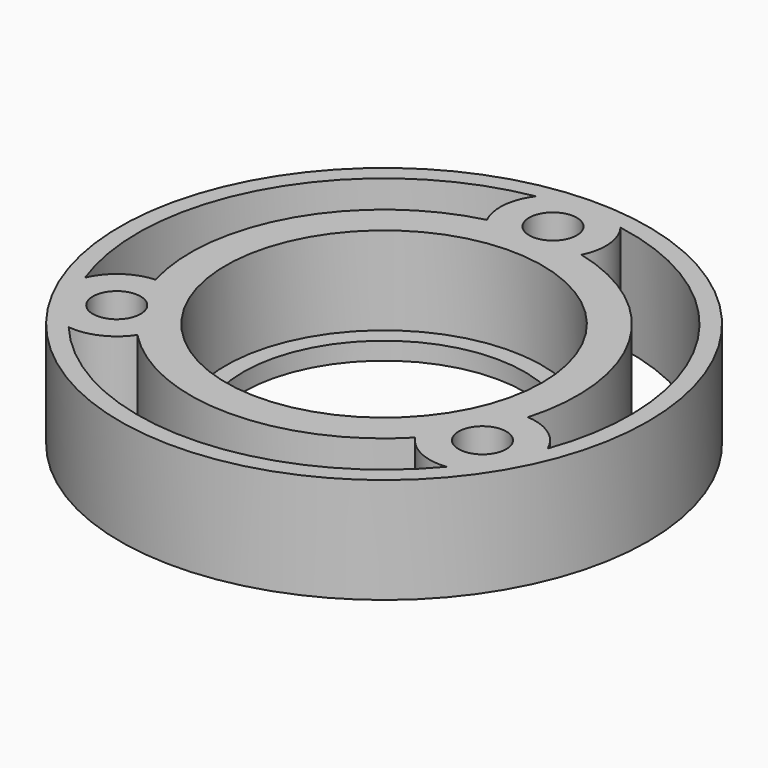
from build123d import *

# Parameters (mm, degrees)
F0_R            = 23.8125
F0_R_2          = 2.15265
F0_R_3          = 12.7
F1_DEPTH        = 9.525
F2_R            = 14.2875
F3_DEPTH        = 7.9375
F5_DEPTH        = 9.525
F5_COPIES_COUNT = 3


# Not quite as in the source:
# - a pattern or mirror of a feature is missing from the dataset's text; its kind, count and spacing are read off the source's solid


with BuildPart() as f1:
    # F0 (on Top) → F1 (new body)
    with BuildSketch(Plane.XY):
        Circle(F0_R)
        with Locations((-16.4977839421, -9.525)):
            Circle(F0_R_2, mode=Mode.SUBTRACT)
        with Locations((16.4977839421, -9.525)):
            Circle(F0_R_2, mode=Mode.SUBTRACT)
        Circle(F0_R_3, mode=Mode.SUBTRACT)
        with Locations((0, 19.05)):
            Circle(F0_R_2, mode=Mode.SUBTRACT)
    extrude(amount=F1_DEPTH)

    # F2 (on face) → F3 (cut)
    with BuildSketch(Plane.XY.offset(9.525)):
        Circle(F2_R)
    extrude(amount=-F3_DEPTH, mode=Mode.SUBTRACT)

    # F4 (on face) → F5 (cut, through all)
    with BuildSketch(Plane.XY.offset(9.525)):
        with BuildLine():
            ThreePointArc((17.0510516982, -14.2552538029), (14.4957458217, -13.8462555599), (12.5315578082, -12.1613718449))
            ThreePointArc((12.5315578082, -12.1613718449), (0, -17.4625), (-12.5315578082, -12.1613718449))
            ThreePointArc((-12.5315578082, -12.1613718449), (-14.4957458217, -13.8462555599), (-17.0510516982, -14.2552538029))
            ThreePointArc((-17.0510516982, -14.2552538029), (0, -22.225), (17.0510516982, -14.2552538029))
        make_face()
    f5 = extrude(amount=-F5_DEPTH, mode=Mode.SUBTRACT)

    # F5_copies: F5 ×3 about axis
    f5_copies_axis = Axis((0, 0, 0), (0, 0, 1))
    for i in range(1, F5_COPIES_COUNT):
        add(f5.rotate(f5_copies_axis, i * 360 / F5_COPIES_COUNT), mode=Mode.SUBTRACT)


solid = f1.part
